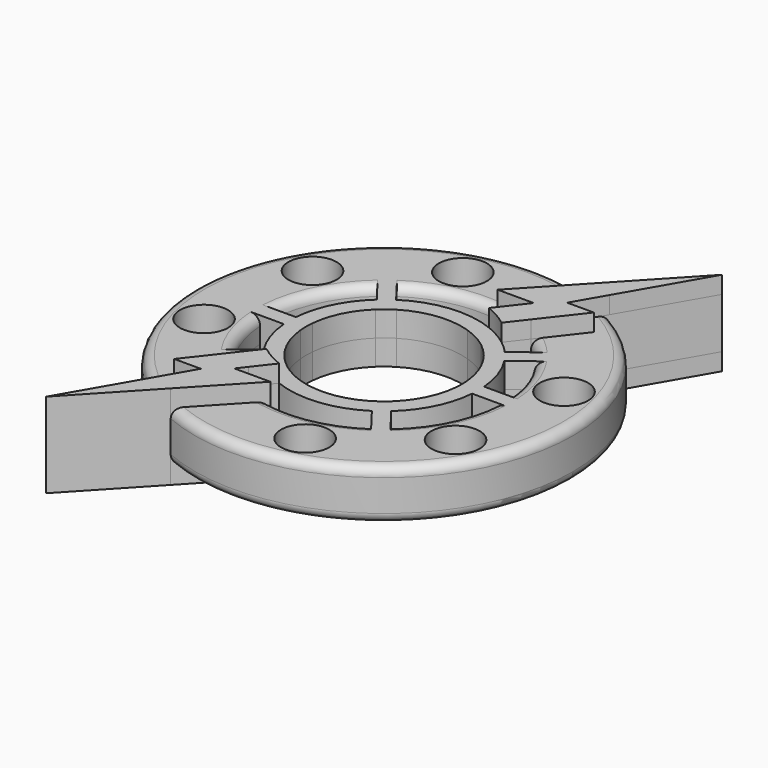
from build123d import *

# Parameters (mm, degrees)
F0_R     = 3.2385
F0_R_2   = 3.2381866017
F1_DEPTH = 3.3909
F2_R     = 1.27
F3_DEPTH = 5.715
F4_DEPTH = 3.3909
F5_R     = 1.27


# Not quite as in the source:
# - a feature names something its author has since deleted; it is built from what else it names


with BuildPart() as f1:
    # F0 (on Top) → F1 (new body, symmetric)
    with BuildSketch(Plane.XY):
        with BuildLine():
            ThreePointArc((9.7360270168, 12.5389554161), (8.2585568463, 13.5577234009), (6.6755407915, 14.4032211724))
            Line((6.6755407915, 14.4032211724), (4.6590682266, 11.8145284824))
            ThreePointArc((4.6590682266, 11.8145284824), (6.2853529091, 11.0355941756), (7.7849274443, 10.0341867975))
            Line((7.7849274443, 10.0341867975), (9.7360270168, 12.5389554161))
        make_face()
        with BuildLine():
            Line((-12.6592947671, 1.016), (-15.8424546394, 1.016))
            ThreePointArc((-15.8424546394, 1.016), (-15.875, 0), (-15.8424546394, -1.016))
            Line((-15.8424546394, -1.016), (-12.6592947671, -1.016))
            ThreePointArc((-12.6592947671, -1.016), (-12.7, 0), (-12.6592947671, 1.016))
        make_face()
        with BuildLine():
            ThreePointArc((-9.7360270168, -12.5389554161), (-8.2585568463, -13.5577234009), (-6.6755407915, -14.4032211724))
            Line((-6.6755407915, -14.4032211724), (-4.6590682266, -11.8145284824))
            ThreePointArc((-4.6590682266, -11.8145284824), (-6.2853529091, -11.0355941756), (-7.7849274443, -10.0341867975))
            Line((-7.7849274443, -10.0341867975), (-9.7360270168, -12.5389554161))
        make_face()
        with BuildLine():
            Line((12.6592947671, -1.016), (15.8424546394, -1.016))
            ThreePointArc((15.8424546394, -1.016), (15.8668615737, -0.5082605632), (15.875, 0))
            ThreePointArc((15.875, 0), (15.8668615737, 0.5082605632), (15.8424546394, 1.016))
            Line((15.8424546394, 1.016), (12.6592947671, 1.016))
            ThreePointArc((12.6592947671, 1.016), (12.6898196114, 0.5084075422), (12.7, 0))
            ThreePointArc((12.7, 0), (12.6898196114, -0.5084075422), (12.6592947671, -1.016))
        make_face()
        with BuildLine():
            ThreePointArc((10.0102182148, 23.3442826254), (11.3750720865, 22.7105203601), (12.7, 21.9970452561))
            Line((12.7, 21.9970452561), (19.05, 32.9955678842))
            Line((19.05, 32.9955678842), (10.0102182148, 23.3442826254))
        make_face()
        with BuildLine():
            Line((-19.05, -32.9955678842), (-10.0102182148, -23.3442826254))
            ThreePointArc((-10.0102182148, -23.3442826254), (-11.3750720865, -22.7105203601), (-12.7, -21.9970452561))
            Line((-12.7, -21.9970452561), (-19.05, -32.9955678842))
        make_face()
        with BuildLine():
            Line((10.3266978221, 17.8863653022), (12.7, 21.9970452561))
            ThreePointArc((12.7, 21.9970452561), (11.3750720865, 22.7105203601), (10.0102182148, 23.3442826254))
            Line((10.0102182148, 23.3442826254), (2.7837893393, 15.6290160252))
            Line((2.7837893393, 15.6290160252), (7.6303786138, 15.6290160252))
            Line((7.6303786138, 15.6290160252), (6.6755407915, 14.4032211724))
            ThreePointArc((6.6755407915, 14.4032211724), (8.2585568463, 13.5577234009), (9.7360270168, 12.5389554161))
            Line((9.7360270168, 12.5389554161), (13.9014134184, 17.8863653022))
            Line((13.9014134184, 17.8863653022), (10.3266978221, 17.8863653022))
        make_face()
        with BuildLine():
            ThreePointArc((-12.7, -21.9970452561), (-11.3750720865, -22.7105203601), (-10.0102182148, -23.3442826254))
            Line((-10.0102182148, -23.3442826254), (-2.7837893393, -15.6290160252))
            Line((-2.7837893393, -15.6290160252), (-7.6303786138, -15.6290160252))
            Line((-7.6303786138, -15.6290160252), (-6.6755407915, -14.4032211724))
            ThreePointArc((-6.6755407915, -14.4032211724), (-8.2585568463, -13.5577234009), (-9.7360270168, -12.5389554161))
            Line((-9.7360270168, -12.5389554161), (-13.9014134184, -17.8863653022))
            Line((-13.9014134184, -17.8863653022), (-10.3266978221, -17.8863653022))
            Line((-10.3266978221, -17.8863653022), (-12.7, -21.9970452561))
        make_face()
        with BuildLine():
            Line((2.7837893393, 15.6290160252), (10.0102182148, 23.3442826254))
            ThreePointArc((10.0102182148, 23.3442826254), (-22.7105203601, 11.3750720865), (-12.7, -21.9970452561))
            Line((-12.7, -21.9970452561), (-10.3266978221, -17.8863653022))
            Line((-10.3266978221, -17.8863653022), (-13.9014134184, -17.8863653022))
            Line((-13.9014134184, -17.8863653022), (-9.7360270168, -12.5389554161))
            ThreePointArc((-9.7360270168, -12.5389554161), (-10.8932687061, -11.5478275834), (-11.9501626947, -10.450322319))
            Line((-11.9501626947, -10.450322319), (-13.2153651543, -11.4211463116))
            Line((-13.2153651543, -11.4211463116), (-14.4523683781, -9.8090523241))
            Line((-14.4523683781, -9.8090523241), (-13.1871659184, -8.8382283315))
            ThreePointArc((-13.1871659184, -8.8382283315), (-15.0325158057, -5.1028515117), (-15.8424546394, -1.016))
            Line((-15.8424546394, -1.016), (-21.3218769546, -1.016))
            Line((-21.3218769546, -1.016), (-21.3218769546, 1.016))
            Line((-21.3218769546, 1.016), (-15.8424546394, 1.016))
            ThreePointArc((-15.8424546394, 1.016), (-14.2378547718, 7.0213329572), (-10.450322319, 11.9501626947))
            Line((-10.450322319, 11.9501626947), (-11.169207399, 12.887031971))
            Line((-11.169207399, 12.887031971), (-9.5571134115, 14.1240351948))
            Line((-9.5571134115, 14.1240351948), (-8.8382283315, 13.1871659184))
            ThreePointArc((-8.8382283315, 13.1871659184), (-3.2641562254, 15.5357944482), (2.7837893393, 15.6290160252))
        make_face()
        with Locations((-19.93429424, -5.3413780433)):
            Circle(F0_R, mode=Mode.SUBTRACT)
        with Locations((-17.8725992706, 10.31875)):
            Circle(F0_R, mode=Mode.SUBTRACT)
        with Locations((-5.3413780433, 19.93429424)):
            Circle(F0_R, mode=Mode.SUBTRACT)
        with BuildLine():
            ThreePointArc((-10.0102182148, -23.3442826254), (13.9803515218, -21.2063615768), (25.4, 0))
            ThreePointArc((25.4, 0), (21.9970452561, 12.7), (12.7, 21.9970452561))
            Line((12.7, 21.9970452561), (10.3266978221, 17.8863653022))
            Line((10.3266978221, 17.8863653022), (13.9014134184, 17.8863653022))
            Line((13.9014134184, 17.8863653022), (9.7360270168, 12.5389554161))
            ThreePointArc((9.7360270168, 12.5389554161), (10.8932687061, 11.5478275834), (11.9501626947, 10.450322319))
            Line((11.9501626947, 10.450322319), (13.5921580143, 11.7102696419))
            Line((13.5921580143, 11.7102696419), (14.2106596262, 10.9042226482))
            Line((14.2106596262, 10.9042226482), (14.8291612381, 10.0981756544))
            Line((14.8291612381, 10.0981756544), (13.1871659184, 8.8382283315))
            ThreePointArc((13.1871659184, 8.8382283315), (15.0325158057, 5.1028515117), (15.8424546394, 1.016))
            Line((15.8424546394, 1.016), (21.3218769546, 1.016))
            Line((21.3218769546, 1.016), (21.3218769546, -1.016))
            Line((21.3218769546, -1.016), (15.8424546394, -1.016))
            ThreePointArc((15.8424546394, -1.016), (14.2378547718, -7.0213329572), (10.450322319, -11.9501626947))
            Line((10.450322319, -11.9501626947), (11.0788852097, -12.7693218023))
            Line((11.0788852097, -12.7693218023), (9.4667912222, -14.006325026))
            Line((9.4667912222, -14.006325026), (8.8382283315, -13.1871659184))
            ThreePointArc((8.8382283315, -13.1871659184), (3.2641562254, -15.5357944482), (-2.7837893393, -15.6290160252))
            Line((-2.7837893393, -15.6290160252), (-10.0102182148, -23.3442826254))
        make_face()
        with Locations((5.3413780433, -19.93429424)):
            Circle(F0_R, mode=Mode.SUBTRACT)
        with Locations((17.8725992706, -10.31875)):
            Circle(F0_R_2, mode=Mode.SUBTRACT)
        with Locations((19.93429424, 5.3413780433)):
            Circle(F0_R, mode=Mode.SUBTRACT)
        with BuildLine():
            Line((-7.6303786138, -15.6290160252), (-2.7837893393, -15.6290160252))
            ThreePointArc((-2.7837893393, -15.6290160252), (-4.7692111387, -15.1416726326), (-6.6755407915, -14.4032211724))
            Line((-6.6755407915, -14.4032211724), (-7.6303786138, -15.6290160252))
        make_face()
        with BuildLine():
            Line((7.6303786138, 15.6290160252), (2.7837893393, 15.6290160252))
            ThreePointArc((2.7837893393, 15.6290160252), (4.7692111387, 15.1416726326), (6.6755407915, 14.4032211724))
            Line((6.6755407915, 14.4032211724), (7.6303786138, 15.6290160252))
        make_face()
        with BuildLine():
            ThreePointArc((-15.8424546394, -1.016), (-15.875, 0), (-15.8424546394, 1.016))
            Line((-15.8424546394, 1.016), (-21.3218769546, 1.016))
            Line((-21.3218769546, 1.016), (-21.3218769546, -1.016))
            Line((-21.3218769546, -1.016), (-15.8424546394, -1.016))
        make_face()
        with BuildLine():
            Line((-10.4281230454, 1.016), (-12.6592947671, 1.016))
            ThreePointArc((-12.6592947671, 1.016), (-12.7, 0), (-12.6592947671, -1.016))
            Line((-12.6592947671, -1.016), (-10.4281230454, -1.016))
            ThreePointArc((-10.4281230454, -1.016), (-10.4775, 0), (-10.4281230454, 1.016))
        make_face()
        with BuildLine():
            ThreePointArc((-9.4247921773, -8.5125373664), (-8.638429638, -9.3095399128), (-7.7849274443, -10.0341867975))
            Line((-7.7849274443, -10.0341867975), (-6.4191566835, -8.2808474037))
            ThreePointArc((-6.4191566835, -8.2808474037), (-9.173451396, -5.0621927793), (-10.4281230454, -1.016))
            Line((-10.4281230454, -1.016), (-12.6592947671, -1.016))
            ThreePointArc((-12.6592947671, -1.016), (-12.0260126446, -4.0822812093), (-10.6617954011, -6.9004433789))
            Line((-10.6617954011, -6.9004433789), (-9.3677261834, -5.9074691439))
            Line((-9.3677261834, -5.9074691439), (-8.1307229597, -7.5195631314))
            Line((-8.1307229597, -7.5195631314), (-9.4247921773, -8.5125373664))
        make_face()
        with BuildLine():
            ThreePointArc((4.6590682266, 11.8145284824), (-1.2602138837, 12.6373201656), (-6.9004433789, 10.6617954011))
            Line((-6.9004433789, 10.6617954011), (-6.6325914278, 10.3127239422))
            Line((-6.6325914278, 10.3127239422), (-8.2446854153, 9.0757207185))
            Line((-8.2446854153, 9.0757207185), (-8.5125373664, 9.4247921773))
            ThreePointArc((-8.5125373664, 9.4247921773), (-11.3902838175, 5.6170663658), (-12.6592947671, 1.016))
            Line((-12.6592947671, 1.016), (-10.4281230454, 1.016))
            ThreePointArc((-10.4281230454, 1.016), (-9.4110801737, 4.6053855662), (-7.2008654679, 7.6108831789))
            ThreePointArc((-7.2008654679, 7.6108831789), (-6.3782978724, 8.3123596229), (-5.487827499, 8.9253434439))
            ThreePointArc((-5.487827499, 8.9253434439), (-1.2474392729, 10.4029756085), (3.2220816094, 9.9697641071))
            Line((3.2220816094, 9.9697641071), (4.6590682266, 11.8145284824))
        make_face()
        with BuildLine():
            ThreePointArc((9.4247921773, 8.5125373664), (8.638429638, 9.3095399128), (7.7849274443, 10.0341867975))
            Line((7.7849274443, 10.0341867975), (6.4191566835, 8.2808474037))
            ThreePointArc((6.4191566835, 8.2808474037), (9.173451396, 5.0621927793), (10.4281230454, 1.016))
            Line((10.4281230454, 1.016), (12.6592947671, 1.016))
            ThreePointArc((12.6592947671, 1.016), (12.0260126446, 4.0822812094), (10.6617954011, 6.9004433789))
            Line((10.6617954011, 6.9004433789), (9.6041638755, 6.088894166))
            Line((9.6041638755, 6.088894166), (8.3519163253, 7.6892907704))
            Line((8.3519163253, 7.6892907704), (9.4247921773, 8.5125373664))
        make_face()
        with BuildLine():
            ThreePointArc((-4.6590682266, -11.8145284824), (1.2602138837, -12.6373201656), (6.9004433789, -10.6617954011))
            Line((6.9004433789, -10.6617954011), (6.1122448207, -9.6345950411))
            Line((6.1122448207, -9.6345950411), (7.7243388082, -8.3975918174))
            Line((7.7243388082, -8.3975918174), (8.5125373664, -9.4247921773))
            ThreePointArc((8.5125373664, -9.4247921773), (11.3902838175, -5.6170663658), (12.6592947671, -1.016))
            Line((12.6592947671, -1.016), (10.4281230454, -1.016))
            ThreePointArc((10.4281230454, -1.016), (5.7466713161, -8.7609231839), (-3.2220816094, -9.9697641071))
            Line((-3.2220816094, -9.9697641071), (-4.6590682266, -11.8145284824))
        make_face()
        with BuildLine():
            Line((10.4281230454, -1.016), (12.6592947671, -1.016))
            ThreePointArc((12.6592947671, -1.016), (12.6898196114, -0.5084075422), (12.7, 0))
            ThreePointArc((12.7, 0), (12.6898196114, 0.5084075422), (12.6592947671, 1.016))
            Line((12.6592947671, 1.016), (10.4281230454, 1.016))
            ThreePointArc((10.4281230454, 1.016), (10.465148481, 0.5085995683), (10.4775, 0))
            ThreePointArc((10.4775, 0), (10.465148481, -0.5085995683), (10.4281230454, -1.016))
        make_face()
        with BuildLine():
            ThreePointArc((-7.7849274443, -10.0341867975), (-6.2853529091, -11.0355941756), (-4.6590682266, -11.8145284824))
            Line((-4.6590682266, -11.8145284824), (-3.2220816094, -9.9697641071))
            ThreePointArc((-3.2220816094, -9.9697641071), (-4.8940248123, -9.2642607577), (-6.4191566835, -8.2808474037))
            Line((-6.4191566835, -8.2808474037), (-7.7849274443, -10.0341867975))
        make_face()
        with BuildLine():
            ThreePointArc((7.7849274443, 10.0341867975), (6.2853529091, 11.0355941756), (4.6590682266, 11.8145284824))
            Line((4.6590682266, 11.8145284824), (3.2220816094, 9.9697641071))
            ThreePointArc((3.2220816094, 9.9697641071), (4.8940248123, 9.2642607577), (6.4191566835, 8.2808474037))
            Line((6.4191566835, 8.2808474037), (7.7849274443, 10.0341867975))
        make_face()
        with BuildLine():
            ThreePointArc((15.875, 0), (15.8668615737, -0.5082605632), (15.8424546394, -1.016))
            Line((15.8424546394, -1.016), (21.3218769546, -1.016))
            Line((21.3218769546, -1.016), (21.3218769546, 1.016))
            Line((21.3218769546, 1.016), (15.8424546394, 1.016))
            ThreePointArc((15.8424546394, 1.016), (15.8668615737, 0.5082605632), (15.875, 0))
        make_face()
        with BuildLine():
            Line((-6.9004433789, 10.6617954011), (-8.8382283315, 13.1871659184))
            Line((-8.8382283315, 13.1871659184), (-10.450322319, 11.9501626947))
            Line((-10.450322319, 11.9501626947), (-8.5125373664, 9.4247921773))
            ThreePointArc((-8.5125373664, 9.4247921773), (-7.7312701484, 10.0755874217), (-6.9004433789, 10.6617954011))
        make_face()
        with BuildLine():
            Line((6.9004433789, -10.6617954011), (8.8382283315, -13.1871659184))
            Line((8.8382283315, -13.1871659184), (10.450322319, -11.9501626947))
            Line((10.450322319, -11.9501626947), (8.5125373664, -9.4247921773))
            ThreePointArc((8.5125373664, -9.4247921773), (7.7312701484, -10.0755874217), (6.9004433789, -10.6617954011))
        make_face()
        Polygon((6.1122448207, -9.6345950411), (6.9004433789, -10.6617954011), (8.5125373664, -9.4247921773), (7.7243388082, -8.3975918174), align=None)
        with BuildLine():
            ThreePointArc((10.450322319, -11.9501626947), (9.6640876855, -12.5944842771), (8.8382283315, -13.1871659184))
            Line((8.8382283315, -13.1871659184), (9.4667912222, -14.006325026))
            Line((9.4667912222, -14.006325026), (11.0788852097, -12.7693218023))
            Line((11.0788852097, -12.7693218023), (10.450322319, -11.9501626947))
        make_face()
        with BuildLine():
            ThreePointArc((-10.450322319, 11.9501626947), (-9.6640876855, 12.5944842771), (-8.8382283315, 13.1871659184))
            Line((-8.8382283315, 13.1871659184), (-9.5571134115, 14.1240351948))
            Line((-9.5571134115, 14.1240351948), (-11.169207399, 12.887031971))
            Line((-11.169207399, 12.887031971), (-10.450322319, 11.9501626947))
        make_face()
        Polygon((-6.6325914278, 10.3127239422), (-6.9004433789, 10.6617954011), (-8.5125373664, 9.4247921773), (-8.2446854153, 9.0757207185), align=None)
        with BuildLine():
            Line((-10.450322319, 11.9501626947), (-8.8382283315, 13.1871659184))
            ThreePointArc((-8.8382283315, 13.1871659184), (-9.6640876855, 12.5944842771), (-10.450322319, 11.9501626947))
        make_face()
        with BuildLine():
            Line((-8.5125373664, 9.4247921773), (-6.9004433789, 10.6617954011))
            ThreePointArc((-6.9004433789, 10.6617954011), (-7.7312701484, 10.0755874217), (-8.5125373664, 9.4247921773))
        make_face()
        with BuildLine():
            Line((10.450322319, -11.9501626947), (8.8382283315, -13.1871659184))
            ThreePointArc((8.8382283315, -13.1871659184), (9.6640876855, -12.5944842771), (10.450322319, -11.9501626947))
        make_face()
        with BuildLine():
            Line((8.5125373664, -9.4247921773), (6.9004433789, -10.6617954011))
            ThreePointArc((6.9004433789, -10.6617954011), (7.7312701484, -10.0755874217), (8.5125373664, -9.4247921773))
        make_face()
        with BuildLine():
            Line((-13.2153651543, -11.4211463116), (-11.9501626947, -10.450322319))
            ThreePointArc((-11.9501626947, -10.450322319), (-12.5944842771, -9.6640876855), (-13.1871659184, -8.8382283315))
            Line((-13.1871659184, -8.8382283315), (-14.4523683781, -9.8090523241))
            Line((-14.4523683781, -9.8090523241), (-13.2153651543, -11.4211463116))
        make_face()
        with BuildLine():
            ThreePointArc((-13.1871659184, -8.8382283315), (-12.5944842771, -9.6640876855), (-11.9501626947, -10.450322319))
            Line((-11.9501626947, -10.450322319), (-9.4247921773, -8.5125373664))
            ThreePointArc((-9.4247921773, -8.5125373664), (-10.0755874217, -7.7312701484), (-10.6617954011, -6.9004433789))
            Line((-10.6617954011, -6.9004433789), (-13.1871659184, -8.8382283315))
        make_face()
        with BuildLine():
            ThreePointArc((-10.6617954011, -6.9004433789), (-10.0755874217, -7.7312701484), (-9.4247921773, -8.5125373664))
            Line((-9.4247921773, -8.5125373664), (-8.1307229597, -7.5195631314))
            Line((-8.1307229597, -7.5195631314), (-9.3677261834, -5.9074691439))
            Line((-9.3677261834, -5.9074691439), (-10.6617954011, -6.9004433789))
        make_face()
        with BuildLine():
            Line((13.5921580143, 11.7102696419), (11.9501626947, 10.450322319))
            ThreePointArc((11.9501626947, 10.450322319), (12.5944842771, 9.6640876855), (13.1871659184, 8.8382283315))
            Line((13.1871659184, 8.8382283315), (14.8291612381, 10.0981756544))
            Line((14.8291612381, 10.0981756544), (14.2106596262, 10.9042226482))
            Line((14.2106596262, 10.9042226482), (13.5921580143, 11.7102696419))
        make_face()
        with BuildLine():
            ThreePointArc((13.1871659184, 8.8382283315), (12.5944842771, 9.6640876855), (11.9501626947, 10.450322319))
            Line((11.9501626947, 10.450322319), (9.4247921773, 8.5125373664))
            ThreePointArc((9.4247921773, 8.5125373664), (10.0755874217, 7.7312701484), (10.6617954011, 6.9004433789))
            Line((10.6617954011, 6.9004433789), (13.1871659184, 8.8382283315))
        make_face()
        with BuildLine():
            ThreePointArc((10.6617954011, 6.9004433789), (10.0755874217, 7.7312701484), (9.4247921773, 8.5125373664))
            Line((9.4247921773, 8.5125373664), (8.3519163253, 7.6892907704))
            Line((8.3519163253, 7.6892907704), (9.6041638755, 6.088894166))
            Line((9.6041638755, 6.088894166), (10.6617954011, 6.9004433789))
        make_face()
    extrude(amount=F1_DEPTH, both=True)

    # F2
    f2_edges = [f1.edges().sort_by_distance(p)[0] for p in [
        (10.893269, 11.547828, 3.3909),
        (14.237855, -7.021333, 3.3909),
        (1.240565, -15.826453, 3.3909),
        (-15.032516, -5.102852, 3.3909),
        (-14.237855, 7.021333, 3.3909),
        (-1.240565, 15.826453, 3.3909),
        (-1.240565, 15.826453, -3.3909),
        (-14.237855, 7.021333, -3.3909),
        (-15.032516, -5.102852, -3.3909),
        (10.893269, 11.547828, -3.3909),
        (14.237855, -7.021333, -3.3909),
        (1.240565, -15.826453, -3.3909),
    ]]
    fillet(f2_edges, radius=F2_R)

    # F0 (on Top) → F3 (join, symmetric)
    with BuildSketch(Plane.XY):
        with BuildLine():
            Line((10.3266978221, 17.8863653022), (12.7, 21.9970452561))
            ThreePointArc((12.7, 21.9970452561), (11.3750720865, 22.7105203601), (10.0102182148, 23.3442826254))
            Line((10.0102182148, 23.3442826254), (2.7837893393, 15.6290160252))
            Line((2.7837893393, 15.6290160252), (7.6303786138, 15.6290160252))
            Line((7.6303786138, 15.6290160252), (6.6755407915, 14.4032211724))
            ThreePointArc((6.6755407915, 14.4032211724), (8.2585568463, 13.5577234009), (9.7360270168, 12.5389554161))
            Line((9.7360270168, 12.5389554161), (13.9014134184, 17.8863653022))
            Line((13.9014134184, 17.8863653022), (10.3266978221, 17.8863653022))
        make_face()
        with BuildLine():
            ThreePointArc((10.0102182148, 23.3442826254), (11.3750720865, 22.7105203601), (12.7, 21.9970452561))
            Line((12.7, 21.9970452561), (19.05, 32.9955678842))
            Line((19.05, 32.9955678842), (10.0102182148, 23.3442826254))
        make_face()
        with BuildLine():
            ThreePointArc((-12.7, -21.9970452561), (-11.3750720865, -22.7105203601), (-10.0102182148, -23.3442826254))
            Line((-10.0102182148, -23.3442826254), (-2.7837893393, -15.6290160252))
            Line((-2.7837893393, -15.6290160252), (-7.6303786138, -15.6290160252))
            Line((-7.6303786138, -15.6290160252), (-6.6755407915, -14.4032211724))
            ThreePointArc((-6.6755407915, -14.4032211724), (-8.2585568463, -13.5577234009), (-9.7360270168, -12.5389554161))
            Line((-9.7360270168, -12.5389554161), (-13.9014134184, -17.8863653022))
            Line((-13.9014134184, -17.8863653022), (-10.3266978221, -17.8863653022))
            Line((-10.3266978221, -17.8863653022), (-12.7, -21.9970452561))
        make_face()
        with BuildLine():
            Line((-19.05, -32.9955678842), (-10.0102182148, -23.3442826254))
            ThreePointArc((-10.0102182148, -23.3442826254), (-11.3750720865, -22.7105203601), (-12.7, -21.9970452561))
            Line((-12.7, -21.9970452561), (-19.05, -32.9955678842))
        make_face()
        with BuildLine():
            ThreePointArc((9.7360270168, 12.5389554161), (8.2585568463, 13.5577234009), (6.6755407915, 14.4032211724))
            Line((6.6755407915, 14.4032211724), (4.6590682266, 11.8145284824))
            ThreePointArc((4.6590682266, 11.8145284824), (6.2853529091, 11.0355941756), (7.7849274443, 10.0341867975))
            Line((7.7849274443, 10.0341867975), (9.7360270168, 12.5389554161))
        make_face()
        with BuildLine():
            ThreePointArc((-9.7360270168, -12.5389554161), (-8.2585568463, -13.5577234009), (-6.6755407915, -14.4032211724))
            Line((-6.6755407915, -14.4032211724), (-4.6590682266, -11.8145284824))
            ThreePointArc((-4.6590682266, -11.8145284824), (-6.2853529091, -11.0355941756), (-7.7849274443, -10.0341867975))
            Line((-7.7849274443, -10.0341867975), (-9.7360270168, -12.5389554161))
        make_face()
    extrude(amount=F3_DEPTH, both=True)

    # F0 (on Top) → F4 (join, symmetric)
    with BuildSketch(Plane.XY):
        with BuildLine():
            ThreePointArc((4.6590682266, 11.8145284824), (-1.2602138837, 12.6373201656), (-6.9004433789, 10.6617954011))
            Line((-6.9004433789, 10.6617954011), (-6.6325914278, 10.3127239422))
            Line((-6.6325914278, 10.3127239422), (-8.2446854153, 9.0757207185))
            Line((-8.2446854153, 9.0757207185), (-8.5125373664, 9.4247921773))
            ThreePointArc((-8.5125373664, 9.4247921773), (-11.3902838175, 5.6170663658), (-12.6592947671, 1.016))
            Line((-12.6592947671, 1.016), (-10.4281230454, 1.016))
            ThreePointArc((-10.4281230454, 1.016), (-9.4110801737, 4.6053855662), (-7.2008654679, 7.6108831789))
            ThreePointArc((-7.2008654679, 7.6108831789), (-6.3782978724, 8.3123596229), (-5.487827499, 8.9253434439))
            ThreePointArc((-5.487827499, 8.9253434439), (-1.2474392729, 10.4029756085), (3.2220816094, 9.9697641071))
            Line((3.2220816094, 9.9697641071), (4.6590682266, 11.8145284824))
        make_face()
        with BuildLine():
            ThreePointArc((-7.7849274443, -10.0341867975), (-6.2853529091, -11.0355941756), (-4.6590682266, -11.8145284824))
            Line((-4.6590682266, -11.8145284824), (-3.2220816094, -9.9697641071))
            ThreePointArc((-3.2220816094, -9.9697641071), (-4.8940248123, -9.2642607577), (-6.4191566835, -8.2808474037))
            Line((-6.4191566835, -8.2808474037), (-7.7849274443, -10.0341867975))
        make_face()
        with BuildLine():
            ThreePointArc((9.4247921773, 8.5125373664), (8.638429638, 9.3095399128), (7.7849274443, 10.0341867975))
            Line((7.7849274443, 10.0341867975), (6.4191566835, 8.2808474037))
            ThreePointArc((6.4191566835, 8.2808474037), (9.173451396, 5.0621927793), (10.4281230454, 1.016))
            Line((10.4281230454, 1.016), (12.6592947671, 1.016))
            ThreePointArc((12.6592947671, 1.016), (12.0260126446, 4.0822812094), (10.6617954011, 6.9004433789))
            Line((10.6617954011, 6.9004433789), (9.6041638755, 6.088894166))
            Line((9.6041638755, 6.088894166), (8.3519163253, 7.6892907704))
            Line((8.3519163253, 7.6892907704), (9.4247921773, 8.5125373664))
        make_face()
        with BuildLine():
            ThreePointArc((7.7849274443, 10.0341867975), (6.2853529091, 11.0355941756), (4.6590682266, 11.8145284824))
            Line((4.6590682266, 11.8145284824), (3.2220816094, 9.9697641071))
            ThreePointArc((3.2220816094, 9.9697641071), (4.8940248123, 9.2642607577), (6.4191566835, 8.2808474037))
            Line((6.4191566835, 8.2808474037), (7.7849274443, 10.0341867975))
        make_face()
        with BuildLine():
            ThreePointArc((-9.4247921773, -8.5125373664), (-8.638429638, -9.3095399128), (-7.7849274443, -10.0341867975))
            Line((-7.7849274443, -10.0341867975), (-6.4191566835, -8.2808474037))
            ThreePointArc((-6.4191566835, -8.2808474037), (-9.173451396, -5.0621927793), (-10.4281230454, -1.016))
            Line((-10.4281230454, -1.016), (-12.6592947671, -1.016))
            ThreePointArc((-12.6592947671, -1.016), (-12.0260126446, -4.0822812093), (-10.6617954011, -6.9004433789))
            Line((-10.6617954011, -6.9004433789), (-9.3677261834, -5.9074691439))
            Line((-9.3677261834, -5.9074691439), (-8.1307229597, -7.5195631314))
            Line((-8.1307229597, -7.5195631314), (-9.4247921773, -8.5125373664))
        make_face()
    extrude(amount=F4_DEPTH, both=True)

    # F5
    f5_edges = [f1.edges().sort_by_distance(p)[0] for p in [
        (-10.893269, -11.547828, 3.3909),
        (15.032516, 5.102852, 3.3909),
        (-10.893269, -11.547828, -3.3909),
        (15.032516, 5.102852, -3.3909),
        (22.71052, -11.375072, -3.3909),
        (-22.71052, 11.375072, -3.3909),
        (-22.71052, 11.375072, 3.3909),
        (22.71052, -11.375072, 3.3909),
    ]]
    fillet(f5_edges, radius=F5_R)


solid = f1.part
